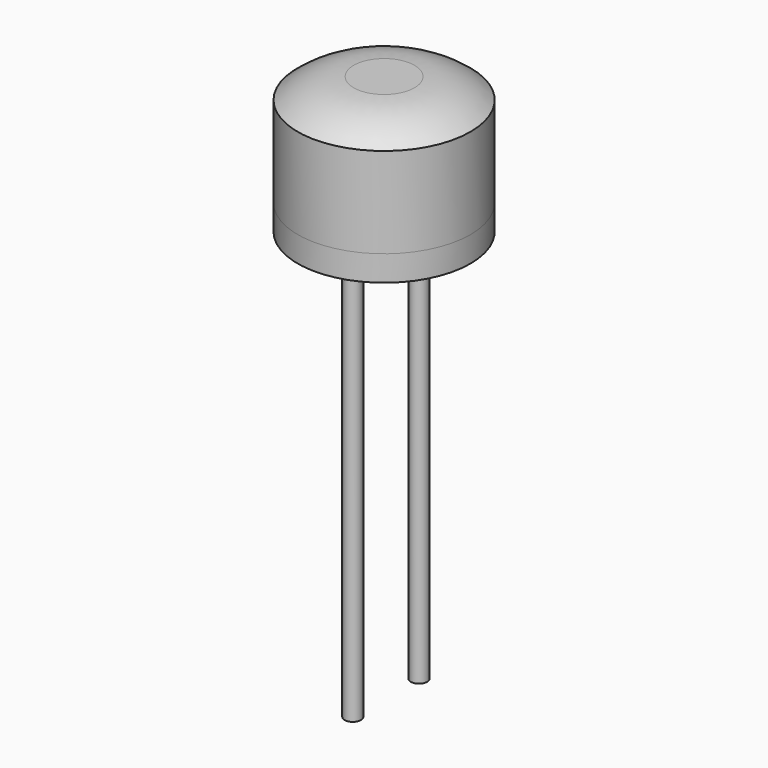
from build123d import *

# Parameters (mm, degrees)
F0_R      = 2.667
F1_DEPTH  = 0.7874
F2_W      = 3.048
F2_H      = 3.81
F3_DEPTH  = 1.905
F4_DEPTH  = 2.794
F5_R      = 1.3827736849
F6_DEPTH  = 0.0254
F7_DEPTH  = 0.635
F9_R      = 0.254
F10_DEPTH = 12.7


# Not quite as in the source:
# - a fillet or chamfer that OpenCascade refuses, or shapes differently, is made with other operations: its cross-section is extruded or revolved along the edge and cut away or added


with BuildPart() as f1:
    # F0 (on Top) → F1 (new body)
    with BuildSketch(Plane.XY):
        Circle(F0_R)
    extrude(amount=-F1_DEPTH)


with BuildPart() as f3:
    # F2 (on face) → F3 (new body)
    with BuildSketch(Plane.XY):
        Rectangle(F2_W, F2_H)
    extrude(amount=F3_DEPTH)

    # F5 (on face) → F6 (cut)
    with BuildSketch(Plane.XY.offset(1.905)):
        Circle(F5_R)
    extrude(amount=-F6_DEPTH, mode=Mode.SUBTRACT)


with BuildPart() as f4:
    # F4 (new): a face of the model
    f4_faces = [f1.part.faces().sort_by_distance(p)[0] for p in [
        (0, 0, 0),
    ]]
    extrude(f4_faces, amount=F4_DEPTH)


with BuildPart() as f7:
    # F7 (new): a face of the model
    f7_faces = [f4.part.faces().sort_by_distance(p)[0] for p in [
        (0, 0, 2.794),
    ]]
    extrude(f7_faces, amount=F7_DEPTH)

    # F8: fillet of radius 2.667 on 1 edges, made by hand

    # F8_s1 → F8_t2 (revolve, cut)
    with BuildSketch(Plane.XZ):
        with BuildLine():
            ThreePointArc((2.667, 2.794), (1.8598156688, 3.2652212247), (0.9396132454, 3.429))
            Line((0.9396132454, 3.429), (0.9396132454, 3.48234))
            Line((0.9396132454, 3.48234), (2.667, 3.48234))
            Line((2.667, 3.48234), (2.72034, 3.429))
            ThreePointArc((2.72034, 3.429), (2.72034, 3.1115), (2.7015477351, 2.83464))
            Line((2.7015477351, 2.83464), (2.667, 2.794))
        make_face()
    revolve(axis=Axis((0, 0, 3.429), (0, 0, 1)), mode=Mode.SUBTRACT)


with BuildPart() as f10:
    # F9 (on face) → F10 (new body)
    with BuildSketch(Plane(origin=(0, 0, -0.7874), x_dir=(1, 0, 0), z_dir=(0, 0, -1))):
        with Locations((0, 1.2091086246)):
            Circle(F9_R)
    extrude(amount=F10_DEPTH)


with BuildPart() as f10b:
    # F9 (on face) → F10, piece 2 (new body)
    with BuildSketch(Plane(origin=(0, 0, -0.7874), x_dir=(1, 0, 0), z_dir=(0, 0, -1))):
        with Locations((0, -1.3476019958)):
            Circle(F9_R)
    extrude(amount=F10_DEPTH)


solid = Compound([f1.part, f3.part, f4.part, f7.part, f10.part, f10b.part])
